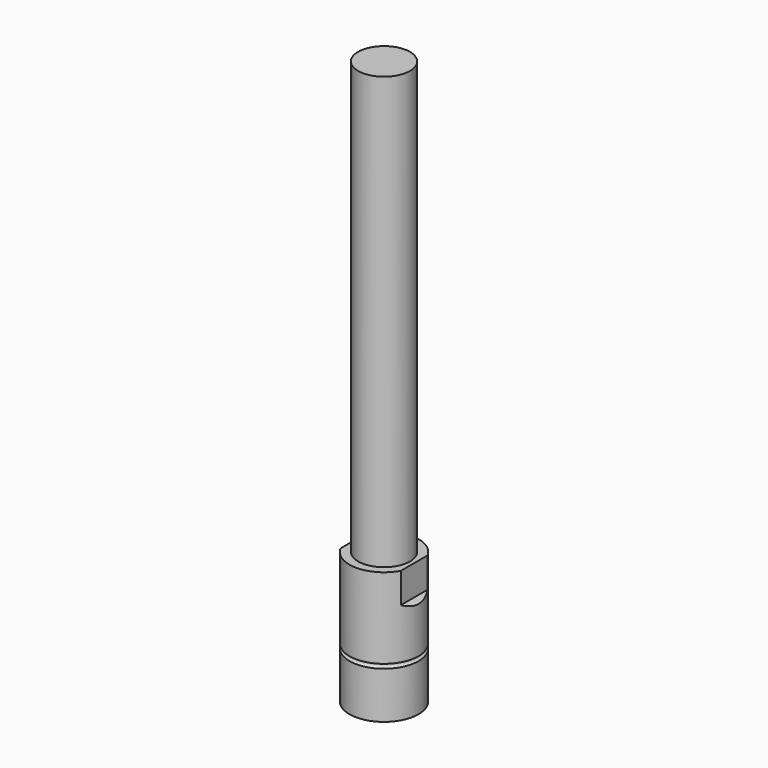
from build123d import *

# Parameters (mm, degrees)
F2_W     = 19.6017324924
F2_H     = 37.1457748115
F2_W_2   = 14
F2_H_2   = 30
F3_DEPTH = 8
F4_SIZE  = 0.99999


# Not quite as in the source:
# - a fillet or chamfer is up to 0.001 mm smaller than in the source, because OpenCascade refuses the exact size


with BuildPart() as f1:
    # F0 (on Front) → F1 (revolve)
    with BuildSketch(Plane.XZ):
        with BuildLine():
            Line((2.9315422289, 21.0469197482), (2.9315422289, 0))
            Line((2.9315422289, 0), (8, 0))
            Line((8, 0), (8, 10.8380244002))
            ThreePointArc((8, 10.8380244002), (7.5, 11.3380244002), (8, 11.8380244002))
            Line((8, 11.8380244002), (8, 30.5))
            Line((8, 30.5), (6, 30.5))
            Line((6, 30.5), (6, 130.5))
            Line((6, 130.5), (0, 130.5))
            Line((0, 130.5), (0, 30.5))
            Line((0, 30.5), (0, 21.0469197482))
            Line((0, 21.0469197482), (2.9315422289, 21.0469197482))
        make_face()
    revolve(axis=Axis((0, 0, 80.5), (0, 0, 1)))

    # F2 (on face) → F3 (cut)
    with BuildSketch(Plane.XY.offset(30.5)):
        Rectangle(F2_W, F2_H)
        Rectangle(F2_W_2, F2_H_2, mode=Mode.SUBTRACT)
    extrude(amount=-F3_DEPTH, mode=Mode.SUBTRACT)

    # F4 (size 1 in the source; OpenCascade refuses exactly that, so slightly less here)
    f4_edges = [f1.edges().sort_by_distance(p)[0] for p in [
        (-7, 0, 22.5),
        (7, 0, 22.5),
    ]]
    chamfer(f4_edges, length=F4_SIZE)


solid = f1.part
